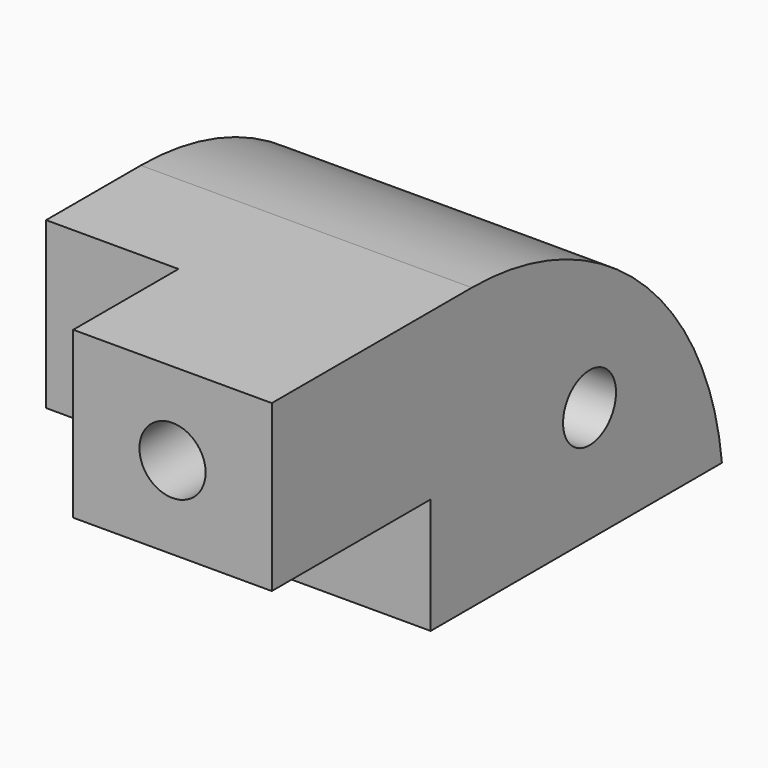
from build123d import *

# Parameters (mm, degrees)
F0_W        = 127
F0_H        = 215.9
F1_DEPTH    = 107.95
F2_W        = 50.4830591381
F2_H        = 107.95
F3_DEPTH    = 50.8
F4_W        = 76.2
F4_H        = 44.45
F5_DEPTH    = 76.2
F8_T1_DEPTH = 726.8985851792
F6_R        = 12.7
F9_DEPTH    = 215.901
F7_R        = 12.7
F10_DEPTH   = 127
F11_W       = 25.4
F11_H       = 44.45
F12_DEPTH   = 50.8


# Not quite as in the source:
# - a fillet or chamfer that OpenCascade refuses, or shapes differently, is made with other operations: its cross-section is extruded or revolved along the edge and cut away or added


with BuildPart() as f1:
    # F0 (on Top) → F1 (new body)
    with BuildSketch(Plane.XY):
        with Locations((-16.8368311822, 57.4669408619)):
            Rectangle(F0_W, F0_H)
    extrude(amount=F1_DEPTH)

    # F2 (on face) → F3 (cut)
    with BuildSketch(Plane(origin=(-80.3368311822, 0, 0), x_dir=(0, -1, 0), z_dir=(-1, 0, 0))):
        with Locations((25.241529569, 53.975)):
            Rectangle(F2_W, F2_H)
    extrude(amount=-F3_DEPTH, mode=Mode.SUBTRACT)

    # F4 (on face) → F5 (cut)
    with BuildSketch(Plane.XZ.offset(50.4830591381)):
        with Locations((8.5631688178, 22.225)):
            Rectangle(F4_W, F4_H)
    extrude(amount=-F5_DEPTH, mode=Mode.SUBTRACT)

    # F8: fillet of radius 120.65 on 1 edges, made by hand

    # F8_s2 → F8_t1 (cut)
    with BuildSketch(Plane.YZ.offset(-380.2861237718)):
        with BuildLine():
            ThreePointArc((165.4169408619, 0), (126.1347067484, 76.9902377631), (45.4372238261, 107.95))
            Line((45.4372238261, 107.95), (165.4169408619, 107.95))
            Line((165.4169408619, 107.95), (165.4169408619, 0))
        make_face()
    extrude(amount=F8_T1_DEPTH, mode=Mode.SUBTRACT)

    # F6 (on face) → F9 (cut, through all)
    with BuildSketch(Plane.XZ.offset(50.4830591381)):
        with Locations((8.5631688178, 76.2)):
            Circle(F6_R)
    extrude(amount=-F9_DEPTH, mode=Mode.SUBTRACT)

    # F7 (on face) → F10 (cut)
    with BuildSketch(Plane.YZ.offset(46.6631688178)):
        with Locations((101.9169408619, 44.45)):
            Circle(F7_R)
    extrude(amount=-F10_DEPTH, mode=Mode.SUBTRACT)

    # F11 (on face) → F12 (cut)
    with BuildSketch(Plane(origin=(-80.3368311822, 0, 0), x_dir=(0, -1, 0), z_dir=(-1, 0, 0))):
        with Locations((-12.7, 22.225)):
            Rectangle(F11_W, F11_H)
    extrude(amount=-F12_DEPTH, mode=Mode.SUBTRACT)


solid = f1.part
